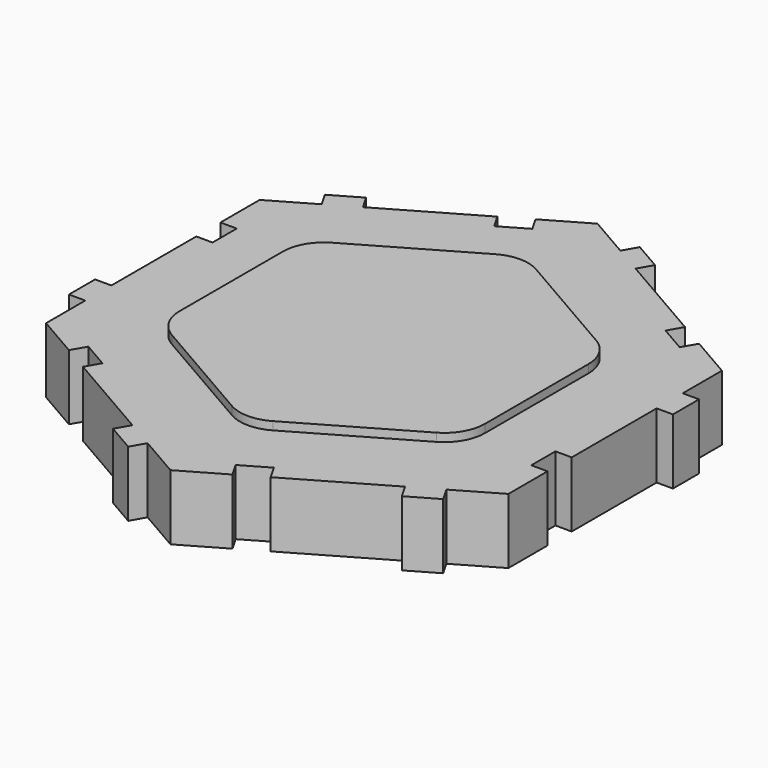
from build123d import *

# Parameters (mm, degrees)
F0_W     = 2
F0_H     = 4
F1_DEPTH = 8
F2_DEPTH = 9
F3_T     = -2
F4_R     = 5
F5_R     = 5
F6_W     = 8.62
F6_H     = 2
F7_DEPTH = 6


with BuildPart() as f1:
    # F0 (on Top) → F1 (new body)
    with BuildSketch(Plane.XY):
        Polygon((-23.121336045, 19.3491095896), (-19.6572344299, 21.3491095896), (-20.6572344299, 23.0811603972), (-24.121336045, 21.0811603972), align=None)
        Polygon((-7.4004464167, 26.1161683716), (-26.3174884677, 15.1944090512), (-26.3174884677, 10.3491095896), (-26.3174884677, 6.6491095896), (-26.3174884677, -15.1944090512), (-22.121336045, -17.617058782), (-18.917042051, -19.467058782), (0, -30.3888181024), (4.1961524227, -27.9661683716), (7.4004464167, -26.1161683716), (26.3174884677, -15.1944090512), (26.3174884677, -10.3491095896), (26.3174884677, -6.6491095896), (26.3174884677, 15.1944090512), (22.121336045, 17.617058782), (18.917042051, 19.467058782), (0, 30.3888181024), (-4.1961524227, 27.9661683716), align=None)
        Polygon((0, -21.59), (-18.6974884677, -10.795), (-18.6974884677, 10.795), (0, 21.59), (18.6974884677, 10.795), (18.6974884677, -10.795), align=None, mode=Mode.SUBTRACT)
        Polygon((-5.1961524227, -29.6982191792), (-8.6602540378, -27.6982191792), (-9.6602540378, -29.4302699868), (-6.1961524227, -31.4302699868), align=None)
        with Locations((29.3174884677, 8.3491095896)):
            Rectangle(F0_W, F0_H)
        with Locations((-29.3174884677, -8.3491095896)):
            Rectangle(F0_W, F0_H)
        Polygon((-26.3174884677, -15.1944090512), (-26.3174884677, 6.6491095896), (-28.3174884677, 6.6491095896), (-28.3174884677, -6.3491095896), (-28.3174884677, -10.3491095896), (-28.3174884677, -16.3491095896), (-23.121336045, -19.3491095896), (-22.121336045, -17.617058782), align=None)
        Polygon((-26.3174884677, 10.3491095896), (-26.3174884677, 15.1944090512), (-7.4004464167, 26.1161683716), (-8.4004464167, 27.8482191792), (-19.6572344299, 21.3491095896), (-23.121336045, 19.3491095896), (-28.3174884677, 16.3491095896), (-28.3174884677, 10.3491095896), align=None)
        Polygon((0, -30.3888181024), (-18.917042051, -19.467058782), (-19.917042051, -21.1991095896), (-8.6602540378, -27.6982191792), (-5.1961524227, -29.6982191792), (0, -32.6982191792), (5.1961524227, -29.6982191792), (4.1961524227, -27.9661683716), align=None)
        Polygon((28.3174884677, -10.3491095896), (26.3174884677, -10.3491095896), (26.3174884677, -15.1944090512), (7.4004464167, -26.1161683716), (8.4004464167, -27.8482191792), (19.6572344299, -21.3491095896), (23.121336045, -19.3491095896), (28.3174884677, -16.3491095896), align=None)
        Polygon((23.121336045, -19.3491095896), (19.6572344299, -21.3491095896), (20.6572344299, -23.0811603972), (24.121336045, -21.0811603972), align=None)
        Polygon((-5.1961524227, 29.6982191792), (-4.1961524227, 27.9661683716), (0, 30.3888181024), (18.917042051, 19.467058782), (19.917042051, 21.1991095896), (8.6602540378, 27.6982191792), (5.1961524227, 29.6982191792), (0, 32.6982191792), align=None)
        Polygon((6.1961524227, 31.4302699868), (5.1961524227, 29.6982191792), (8.6602540378, 27.6982191792), (9.6602540378, 29.4302699868), align=None)
        Polygon((23.121336045, 19.3491095896), (22.121336045, 17.617058782), (26.3174884677, 15.1944090512), (26.3174884677, -6.6491095896), (28.3174884677, -6.6491095896), (28.3174884677, 6.3491095896), (28.3174884677, 10.3491095896), (28.3174884677, 16.3491095896), align=None)
    extrude(amount=F1_DEPTH)

    # F0 (on Top) → F2 (join)
    with BuildSketch(Plane.XY):
        Polygon((-18.6974884677, 10.795), (-18.6974884677, -10.795), (0, -21.59), (18.6974884677, -10.795), (18.6974884677, 10.795), (0, 21.59), align=None)
    extrude(amount=F2_DEPTH)

    # F3: a shell. OpenCascade refuses it in one call, so the cavity is built on its own and cut out:
    # the body offset inwards by the wall thickness, plus a prism from it out through each open face.
    f3_core = offset(f1.part, amount=F3_T, kind=Kind.INTERSECTION, mode=Mode.PRIVATE)
    f3_exits = [f3_core.faces().sort_by_distance(p)[0] for p in [
        (0, 0, 2),
    ]]
    add(f3_core, mode=Mode.SUBTRACT)
    extrude(f3_exits, amount=-F3_T, mode=Mode.SUBTRACT)

    # F4
    f4_edges = [f1.edges().sort_by_distance(p)[0] for p in [
        (-18.697488, 10.795, 8.5),
        (-18.697488, -10.795, 8.5),
        (0, -21.59, 8.5),
        (18.697488, -10.795, 8.5),
        (18.697488, 10.795, 8.5),
        (0, 21.59, 8.5),
    ]]
    fillet(f4_edges, radius=F4_R)

    # F5
    f5_edges = [f1.edges().sort_by_distance(p)[0] for p in [
        (16.697488, -9.640299, 6.5),
        (0, -19.280599, 6.5),
        (-16.697488, -9.640299, 6.5),
        (-16.697488, 9.640299, 6.5),
        (0, 19.280599, 6.5),
        (16.697488, 9.640299, 6.5),
    ]]
    fillet(f5_edges, radius=F5_R)

    # F6 (on face) → F7 (join)
    with BuildSketch(Plane(origin=(0, 0, 6), x_dir=(1, 0, 0), z_dir=(0, 0, -1))):
        Polygon((15.2029661558, 21.6113814999), (13.4611243361, 22.6170343434), (8.3950167715, 15.6640247696), (10.0114517622, 14.4862565748), align=None)
        with Locations((-22.0074884677, 4.1833669636)):
            Rectangle(F6_W, F6_H)
        with Locations((22.0074884677, -0.0066501563)):
            Rectangle(F6_W, F6_H)
        Polygon((-12.5819755408, -13.1710924962), (-16.8919755408, -20.6362314769), (-15.1599247332, -21.6362314769), (-10.8499247332, -14.1710924962), align=None)
    extrude(amount=F7_DEPTH)


solid = f1.part
